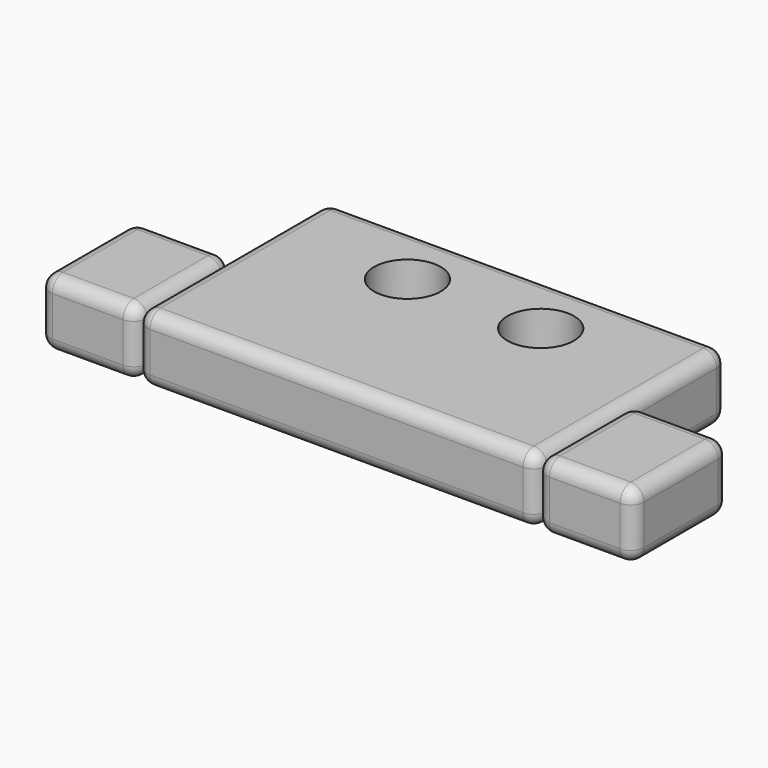
from build123d import *

# Parameters (mm, degrees)
F1_DEPTH     = 10
F0_R         = 5
F2_DEPTH     = 10
F3_R         = 2
F3_2_R       = 2
F3_3_R       = 2
F4_T1_DEPTH  = 17.6
F4_S5_W      = 2.04
F4_S5_H      = 2.04
F4_T6_DEPTH  = 2.04
F4_T9_DEPTH  = 6
F4_T11_DEPTH = 13.9
F4_S15_W     = 2.04
F4_S15_H     = 2.04
F4_T16_DEPTH = 2.04
F4_S21_W     = 2.04
F4_S21_H     = 2.04
F4_T22_DEPTH = 2.04
F4_T26_ANGLE = 90
F4_T28_ANGLE = 90
F4_2_F1_R    = 2


# Not quite as in the source:
# - a fillet or chamfer that OpenCascade refuses, or shapes differently, is made with other operations: its cross-section is extruded or revolved along the edge and cut away or added
# - a feature of the source that left no trace in its solid (it failed there, or was rolled back) is left out


with BuildPart() as f1:
    # F0 (on Top) → F1 (new body)
    with BuildSketch(Plane.XY):
        Polygon((-48.6741693407, -19.0652475223), (-48.6741693407, -1.2101934761), (-63.2741693407, -1.2101934761), (-63.2741693407, -19.1101934761), (-48.6741693407, -19.1101934761), align=None)
    extrude(amount=F1_DEPTH)

    # F3
    f3_edges = [f1.edges().sort_by_distance(p)[0] for p in [
        (-63.274169, -10.160193, 10),
        (-55.974169, -19.110193, 10),
        (-55.974169, -1.210193, 0),
        (-48.674169, -10.160193, 0),
        (-55.974169, -19.110193, 0),
        (-63.274169, -19.110193, 5),
        (-63.274169, -1.210193, 5),
        (-63.274169, -10.160193, 0),
    ]]
    fillet(f3_edges, radius=F3_R)

    # F4: fillet of radius 2 on 2 edges, made by hand

    # F4_s2 → F4_t1 (cut)
    with BuildSketch(Plane.YZ.offset(-61.2741693407)):
        with BuildLine():
            ThreePointArc((-3.2101934761, 10), (-1.7959799137, 9.4142135624), (-1.2101934761, 8))
            Line((-1.2101934761, 8), (-1.1701934761, 8))
            Line((-1.1701934761, 8), (-1.1701934761, 10.04))
            Line((-1.1701934761, 10.04), (-3.2101934761, 10.04))
            Line((-3.2101934761, 10.04), (-3.2101934761, 10))
        make_face()
    extrude(amount=F4_T1_DEPTH, mode=Mode.SUBTRACT)


with BuildPart() as f1b:
    # F0 (on Top) → F1, piece 2 (new body)
    with BuildSketch(Plane.XY):
        Polygon((25.9258306593, -1.2115662456), (11.3258306593, -1.2115662456), (11.3258306593, -19.0652475223), (11.3258306593, -19.1115662456), (25.9258306593, -19.1115662456), align=None)
    extrude(amount=F1_DEPTH)

    # F3#2
    f3_2_edges = [f1b.edges().sort_by_distance(p)[0] for p in [
        (18.625831, -19.111566, 10),
        (18.625831, -1.211566, 10),
        (25.925831, -10.161566, 10),
        (25.925831, -10.161566, 0),
        (25.925831, -1.211566, 5),
        (18.625831, -1.211566, 0),
        (25.925831, -19.111566, 5),
        (18.625831, -19.111566, 0),
    ]]
    fillet(f3_2_edges, radius=F3_2_R)

    # F4#2: fillet of radius 2 on 2 edges, made by hand

    # F4_2_f1
    f4_2_f1_edges = [f1b.edges().sort_by_distance(p)[0] for p in [
        (11.3258306593, -1.2115662456, 5),
        (11.3258306593, -1.7973526832, 0.5857864376),
        (11.3258306593, -1.7973526832, 9.4142135624),
        (11.3258306593, -10.1615662456, 0),
        (11.3258306593, -10.1615662456, 10),
        (11.3258306593, -18.5257798079, 0.5857864376),
        (11.3258306593, -18.5257798079, 9.4142135624),
        (11.3258306593, -19.1115662456, 5),
    ]]
    fillet(f4_2_f1_edges, radius=F4_2_F1_R)


with BuildPart() as f2:
    # F0 (on Top) → F2 (new body)
    with BuildSketch(Plane.XY):
        Polygon((11.3258306593, 16.7347524777), (-48.6741693407, 16.7347524777), (-48.6741693407, -1.2101934761), (-48.6741693407, -19.0652475223), (11.3258306593, -19.0652475223), (11.3258306593, -1.2115662456), align=None)
        with Locations((-28.6741693407, 6.7347524777)):
            Circle(F0_R, mode=Mode.SUBTRACT)
        with Locations((-8.6741693407, 6.7347524777)):
            Circle(F0_R, mode=Mode.SUBTRACT)
    extrude(amount=F2_DEPTH)

    # F3#3
    f3_3_edges = [f2.edges().sort_by_distance(p)[0] for p in [
        (11.325831, -10.161566, 0),
        (-18.674169, 16.734752, 10),
        (11.325831, -1.165248, 10),
        (-48.674169, -1.165248, 10),
        (-18.674169, -19.065248, 10),
        (11.325831, 16.734752, 5),
        (-48.674169, 16.734752, 5),
        (-18.674169, -19.065248, 0),
        (-18.674169, 16.734752, 0),
        (-48.674169, -19.065248, 5),
        (-48.674169, -1.165248, 0),
        (11.325831, -19.065248, 5),
        (11.325831, -1.165248, 0),
    ]]
    fillet(f3_3_edges, radius=F3_3_R)


with BuildPart() as f4_tool4:
    # F4_s5 → F4_t6 (new body)
    with BuildSketch(Plane.XY.offset(8)):
        with Locations((-62.2941693407, -2.1901934761)):
            Rectangle(F4_S5_W, F4_S5_H)
    extrude(amount=F4_T6_DEPTH)

    # F4_s7 → F4_t8 (revolve, cut)
    with BuildSketch(Plane(origin=(-61.2741693407, -3.2101934761, 8), x_dir=(0.7071067812, -0.7071067812, 0), z_dir=(-0.7071067812, -0.7071067812, 0))):
        with BuildLine():
            ThreePointArc((0, -2), (2, 0), (0, 2))
            Line((0, 2), (0, -2))
        make_face()
    revolve(axis=Axis((-61.2741693407, -3.2101934761, 8), (0, 0, 1)), mode=Mode.SUBTRACT)


with BuildPart() as f1_1:
    add(f1.part)

    # F4_t3: cut F4_tool4
    add(f4_tool4.part, mode=Mode.SUBTRACT)

    # F4_s10 → F4_t9 (cut)
    with BuildSketch(Plane.XY.offset(2)):
        with BuildLine():
            ThreePointArc((-50.6741693407, -1.2101934761), (-49.2599557784, -1.7959799137), (-48.6741693407, -3.2101934761))
            Line((-48.6741693407, -3.2101934761), (-48.6341693407, -3.2101934761))
            Line((-48.6341693407, -3.2101934761), (-48.6341693407, -1.1701934761))
            Line((-48.6341693407, -1.1701934761), (-50.6741693407, -1.1701934761))
            Line((-50.6741693407, -1.1701934761), (-50.6741693407, -1.2101934761))
        make_face()
        with BuildLine():
            ThreePointArc((-50.6741693407, -19.1101934761), (-49.2599557784, -18.5244070385), (-48.6741693407, -17.1101934761))
            Line((-48.6741693407, -17.1101934761), (-48.6341693407, -17.1101934761))
            Line((-48.6341693407, -17.1101934761), (-48.6341693407, -19.1501934761))
            Line((-48.6341693407, -19.1501934761), (-50.6741693407, -19.1501934761))
            Line((-50.6741693407, -19.1501934761), (-50.6741693407, -19.1101934761))
        make_face()
    extrude(amount=F4_T9_DEPTH, mode=Mode.SUBTRACT)

    # F4_s12 → F4_t11 (cut)
    with BuildSketch(Plane.XZ.offset(3.2101934761)):
        with BuildLine():
            ThreePointArc((-50.6741693407, 10), (-49.2599557784, 9.4142135624), (-48.6741693407, 8))
            Line((-48.6741693407, 8), (-48.6341693407, 8))
            Line((-48.6341693407, 8), (-48.6341693407, 10.04))
            Line((-48.6341693407, 10.04), (-50.6741693407, 10.04))
            Line((-50.6741693407, 10.04), (-50.6741693407, 10))
        make_face()
    extrude(amount=F4_T11_DEPTH, mode=Mode.SUBTRACT)


with BuildPart() as f4_tool14:
    # F4_s15 → F4_t16 (new body)
    with BuildSketch(Plane.XZ.offset(3.2101934761)):
        with Locations((-49.6541693407, 0.98)):
            Rectangle(F4_S15_W, F4_S15_H)
    extrude(amount=-F4_T16_DEPTH)

    # F4_s17 → F4_t18 (revolve, cut)
    with BuildSketch(Plane(origin=(-50.6741693407, -3.2101934761, 2), x_dir=(-0.7071067812, 0, 0.7071067812), z_dir=(-0.7071067812, 0, -0.7071067812))):
        with BuildLine():
            ThreePointArc((0, -2), (2, 0), (0, 2))
            Line((0, 2), (0, -2))
        make_face()
    revolve(axis=Axis((-50.6741693407, -3.2101934761, 2), (0, 1, 0)), mode=Mode.SUBTRACT)


with BuildPart() as f1_2:
    add(f1_1.part)

    # F4_t13: cut F4_tool14
    add(f4_tool14.part, mode=Mode.SUBTRACT)


with BuildPart() as f4_tool20:
    # F4_s21 → F4_t22 (new body)
    with BuildSketch(Plane.XZ.offset(17.1101934761)):
        with Locations((-49.6541693407, 0.98)):
            Rectangle(F4_S21_W, F4_S21_H)
    extrude(amount=F4_T22_DEPTH)

    # F4_s23 → F4_t24 (revolve, cut)
    with BuildSketch(Plane(origin=(-50.6741693407, -17.1101934761, 2), x_dir=(-0.7071067812, 0, 0.7071067812), z_dir=(0.7071067812, 0, 0.7071067812))):
        with BuildLine():
            ThreePointArc((0, -2), (2, 0), (0, 2))
            Line((0, 2), (0, -2))
        make_face()
    revolve(axis=Axis((-50.6741693407, -17.1101934761, 2), (0, -1, 0)), mode=Mode.SUBTRACT)


with BuildPart() as f1_3:
    add(f1_2.part)

    # F4_t19: cut F4_tool20
    add(f4_tool20.part, mode=Mode.SUBTRACT)

    # F4_s25 → F4_t26 (revolve, cut)
    with BuildSketch(Plane.XY.offset(8)):
        with BuildLine():
            ThreePointArc((-48.6741693407, -3.2101934761), (-49.2599557784, -1.7959799137), (-50.6741693407, -1.2101934761))
            Line((-50.6741693407, -1.2101934761), (-50.6741693407, -1.1701934761))
            Line((-50.6741693407, -1.1701934761), (-48.6341693407, -1.1701934761))
            Line((-48.6341693407, -1.1701934761), (-48.6341693407, -3.2101934761))
            Line((-48.6341693407, -3.2101934761), (-48.6741693407, -3.2101934761))
        make_face()
    revolve(axis=Axis((-48.6741693407, -3.2101934761, 8), (1, 0, 0)), revolution_arc=F4_T26_ANGLE, mode=Mode.SUBTRACT)

    # F4_s27 → F4_t28 (revolve, cut)
    with BuildSketch(Plane.XZ.offset(17.1101934761)):
        with BuildLine():
            ThreePointArc((-50.6741693407, 10), (-49.2599557784, 9.4142135624), (-48.6741693407, 8))
            Line((-48.6741693407, 8), (-48.6341693407, 8))
            Line((-48.6341693407, 8), (-48.6341693407, 10.04))
            Line((-48.6341693407, 10.04), (-50.6741693407, 10.04))
            Line((-50.6741693407, 10.04), (-50.6741693407, 10))
        make_face()
    revolve(axis=Axis((-48.6741693407, -17.1101934761, 8), (1, 0, 0)), revolution_arc=F4_T28_ANGLE, mode=Mode.SUBTRACT)


solid = Compound([f1b.part, f2.part, f1_3.part])
